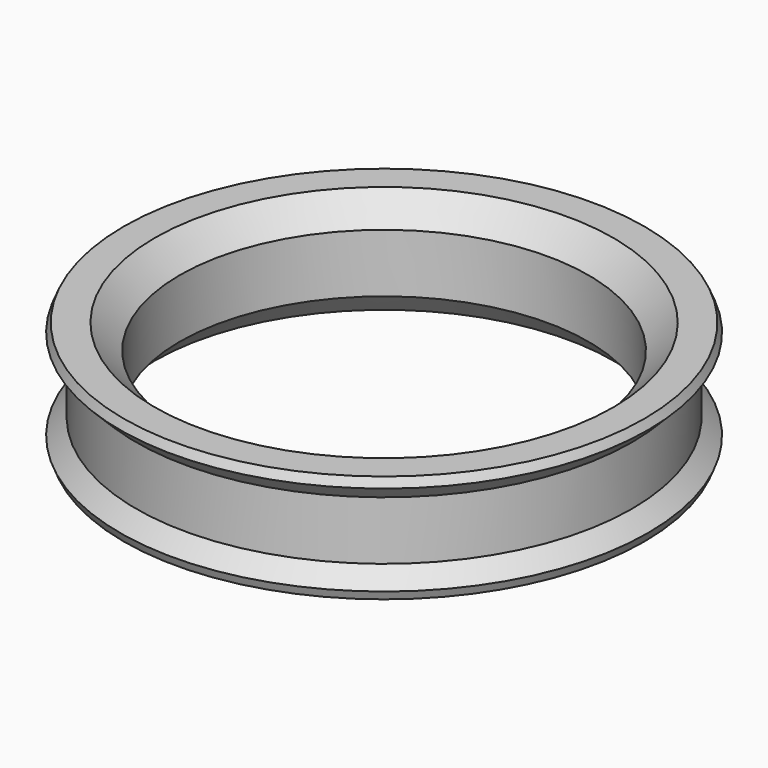
from build123d import *

# Parameters (mm, degrees)
F0_R      = 25.4
F1_DEPTH  = 3
F1_FACE_R = 25.4
F2_DEPTH  = 2.54
F2_TAPER  = -45
F5_R      = 20.955
F6_DEPTH  = 11.081
F7_SIZE   = 2.54


# Not quite as in the source:
# - a fillet or chamfer that OpenCascade refuses, or shapes differently, is made with other operations: its cross-section is extruded or revolved along the edge and cut away or added


with BuildPart() as f1:
    # F0 (on Top) → F1 (new body)
    with BuildSketch(Plane.XY):
        Circle(F0_R)
    extrude(amount=F1_DEPTH)

    # F1_face (on face) → F2 (join)
    with BuildSketch(Plane.XY.offset(3)):
        Circle(F1_FACE_R)
    extrude(amount=F2_DEPTH, taper=F2_TAPER)

    # F3: F1 across plane


with BuildPart() as f1_1:
    add(f1.part)
    add(f1.part.mirror(Plane.XY))

    # F4: chamfer of 1.27 on 2 edges, made by hand

    # F4_s1 → F4_t2 (revolve, cut)
    with BuildSketch(Plane.XZ):
        Polygon((27.0419743879, 4.6419743879), (26.67, 5.54), (27.94, 5.54), align=None)
    revolve(axis=Axis((0, 0, 5.54), (0, 0, -1)), mode=Mode.SUBTRACT)

    # F4_s3 → F4_t4 (revolve, cut)
    with BuildSketch(Plane.XZ):
        Polygon((27.0419743879, -4.6419743879), (26.67, -5.54), (27.94, -5.54), align=None)
    revolve(axis=Axis((0, 0, -5.54), (0, 0, -1)), mode=Mode.SUBTRACT)

    # F5 (on face) → F6 (cut, through all)
    with BuildSketch(Plane(origin=(0, 0, -5.54), x_dir=(1, 0, 0), z_dir=(0, 0, -1))):
        Circle(F5_R)
    extrude(amount=-F6_DEPTH, mode=Mode.SUBTRACT)

    # F7
    f7_edges = [f1_1.edges().sort_by_distance(p)[0] for p in [
        (-20.955, 0, 5.54),
        (-20.955, 0, -5.54),
    ]]
    chamfer(f7_edges, length=F7_SIZE)


solid = f1_1.part
